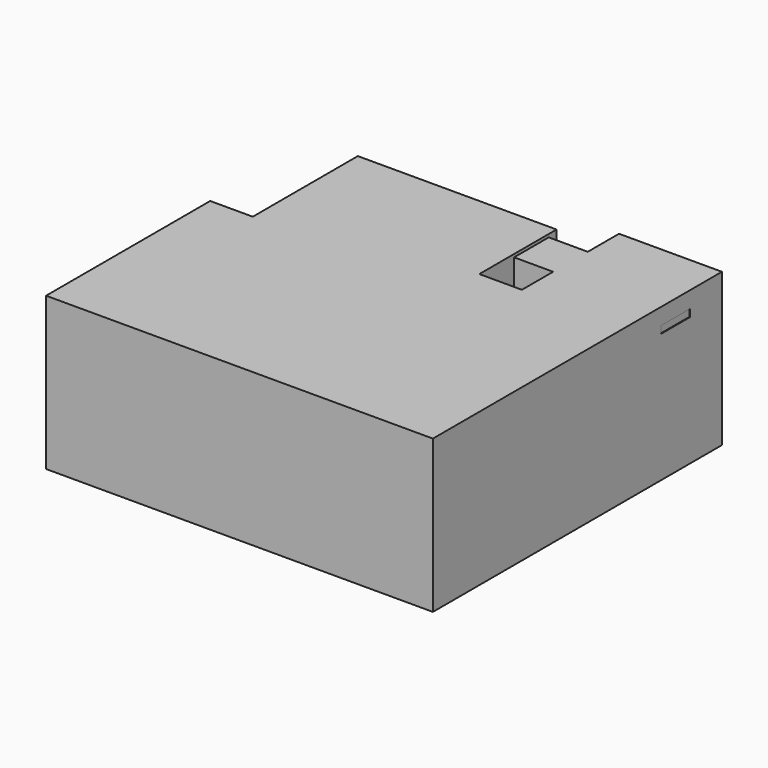
from build123d import *

# Parameters (mm, degrees)
F1_DEPTH  = 910
F2_W      = 600
F2_H      = 1600
F3_DEPTH  = 605
F4_W      = 600
F4_H      = 1600
F5_DEPTH  = 635
F6_W      = 500
F6_H      = 150
F6_H_2    = 350
F7_DEPTH  = 25
F8_W      = 50
F8_H      = 1710
F9_DEPTH  = 2150
F10_W     = 550
F10_H     = 550
F11_DEPTH = 2150
F12_W     = 516.2205696106
F12_H     = 103.4668684006
F13_DEPTH = 10
F14_W     = 5881.225649956
F14_H     = 5462.1144815301
F15_DEPTH = 2150


with BuildPart() as f1:
    # F0 (on Top) → F1 (new body)
    with BuildSketch(Plane.XY):
        Polygon((-1473.1765345304, 1076.0116144037), (-1473.1765345304, -1123.9883855963), (-873.1765345304, -1123.9883855963), (-873.1765345304, 476.0116144037), (1326.8234654696, 476.0116144037), (1326.8234654696, -633.9883855963), (1926.8234654696, -633.9883855963), (1926.8234654696, 1076.0116144037), align=None)
    extrude(amount=F1_DEPTH)

    # F2 (on face) → F3 (join)
    with BuildSketch(Plane.XY.offset(910)):
        with Locations((-1173.1765345304, -323.9883855963)):
            Rectangle(F2_W, F2_H)
    extrude(amount=F3_DEPTH)

    # F4 (on face) → F5 (join)
    with BuildSketch(Plane.XY.offset(1515)):
        Polygon((-1473.1765345304, 476.0116144037), (-873.1765345304, 476.0116144037), (-873.1765345304, 726.0116144037), (1926.8234654696, 726.0116144037), (1926.8234654696, 1076.0116144037), (-1473.1765345304, 1076.0116144037), align=None)
        with Locations((-1173.1765345304, -323.9883855963)):
            Rectangle(F4_W, F4_H)
    extrude(amount=F5_DEPTH)

    # F6 (on face) → F7 (join)
    with BuildSketch(Plane(origin=(0, 0, 1515), x_dir=(1, 0, 0), z_dir=(0, 0, -1))):
        with Locations((250, -651.0116144037)):
            Rectangle(F6_W, F6_H)
        with Locations((250, -901.0116144037)):
            Rectangle(F6_W, F6_H_2)
    extrude(amount=F7_DEPTH)

    # F8 (on face) → F9 (join, through all)
    with BuildSketch(Plane(origin=(0, 0, 0), x_dir=(1, 0, 0), z_dir=(0, 0, -1))):
        with Locations((1951.8234654696, -221.0116144037)):
            Rectangle(F8_W, F8_H)
    extrude(amount=-F9_DEPTH)

    # F10 (on face) → F11 (join, through all)
    with BuildSketch(Plane.XY.offset(2150)):
        with Locations((2251.8234654696, -358.9883855963)):
            Rectangle(F10_W, F10_H)
        with Locations((2251.8234654696, 801.0116144037)):
            Rectangle(F10_W, F10_H)
        Polygon((-1473.1765345304, 1276.0116144037), (-1473.1765345304, 1076.0116144037), (1976.8234654696, 1076.0116144037), (2526.8234654696, 1076.0116144037), (3976.8234654696, 1076.0116144037), (3976.8234654696, 1276.0116144037), align=None)
        Polygon((4246.0098906786, 1276.0116144037), (3976.8234654696, 1276.0116144037), (3976.8234654696, 1076.0116144037), (3976.8234654696, -4014.142036438), (4246.0098906786, -4014.142036438), align=None)
        Polygon((3976.8234654696, -4014.142036438), (-1473.1765345304, -4014.142036438), (-1473.1765345304, -4186.1028671265), (4246.0098906786, -4186.1028671265), (4246.0098906786, -4014.142036438), align=None)
        Polygon((-1473.1765345304, -1123.9883855963), (-1473.1765345304, 1076.0116144037), (-1473.1765345304, 1276.0116144037), (-1635.2157592773, 1276.0116144037), (-1635.2157592773, -4186.1028671265), (-1473.1765345304, -4186.1028671265), (-1473.1765345304, -4014.142036438), align=None)
    extrude(amount=-F11_DEPTH)

    # F12 (on face) → F13 (join)
    with BuildSketch(Plane(origin=(3976.8234654696, 0, 0), x_dir=(0, -1, 0), z_dir=(-1, 0, 0))):
        with Locations((-258.1102848053, 1867.4786686897)):
            Rectangle(F12_W, F12_H)
    extrude(amount=F13_DEPTH)


with BuildPart() as f15:
    # F14 (on face) → F15 (new body, through all)
    with BuildSketch(Plane.XY.offset(2150)):
        with Locations((1305.3970657006, -1455.0456263614)):
            Rectangle(F14_W, F14_H)
    extrude(amount=-F15_DEPTH)

    # F16: cut F1
    add(f1.part, mode=Mode.SUBTRACT)


solid = f15.part
